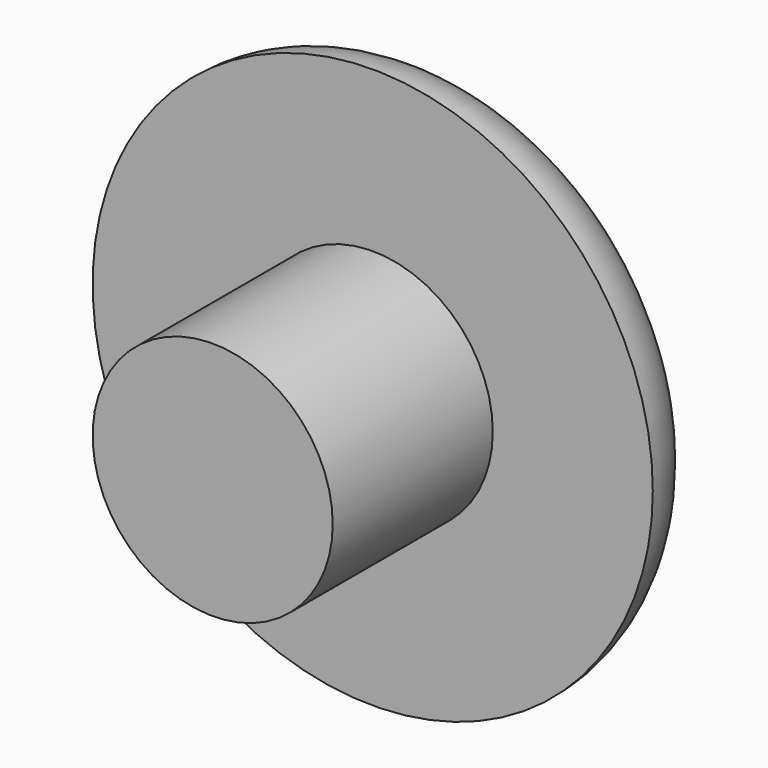
from build123d import *

# Parameters (mm, degrees)
F0_R     = 3
F1_DEPTH = 5
F0_R_2   = 7
F2_DEPTH = 2
F3_R     = 1.99999


# Not quite as in the source:
# - a fillet or chamfer is up to 0.001 mm smaller than in the source, because OpenCascade refuses the exact size


with BuildPart() as f1:
    # F0 (on Front) → F1 (new body)
    with BuildSketch(Plane.XZ):
        Circle(F0_R)
    extrude(amount=F1_DEPTH)

    # F0 (on Front) → F2 (join)
    with BuildSketch(Plane.XZ):
        Circle(F0_R_2)
        Circle(F0_R, mode=Mode.SUBTRACT)
        Circle(F0_R)
    extrude(amount=-F2_DEPTH)

    # F3 (radius 2 in the source; OpenCascade refuses exactly that, so slightly less here)
    f3_edges = [f1.edges().sort_by_distance(p)[0] for p in [
        (-7, 2, 0),
    ]]
    fillet(f3_edges, radius=F3_R)


solid = f1.part
